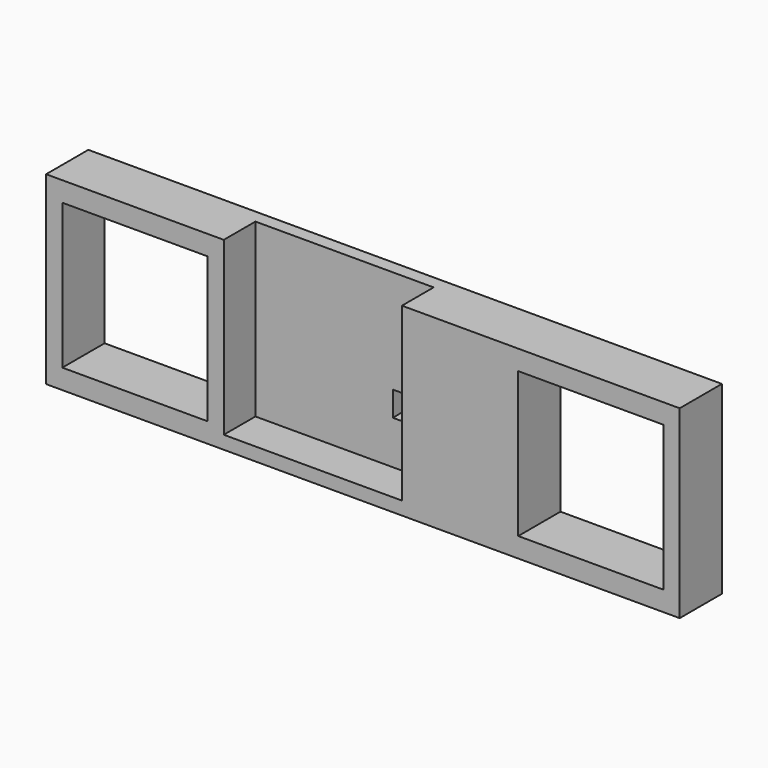
from build123d import *

# Parameters (mm, degrees)
F0_W     = 7.8232
F0_H     = 6.35
F0_W_2   = 69.85
F0_H_2   = 3.175
F0_W_3   = 55.9308
F0_H_3   = 69.85
F0_W_4   = 7.7978
F0_H_4   = 12.7
F0_W_5   = 85.725
F1_DEPTH = 25.4
F0_W_6   = 2.8702
F0_H_5   = 5.1918955931
F0_W_7   = 66.0908
F0_H_6   = 4.9097025247
F0_H_7   = 13.4315382606
F0_W_8   = 16.764
F0_H_8   = 0.762
F2_DEPTH = 6.35


with BuildPart() as f1:
    # F0 (on Front) → F1 (new body)
    with BuildSketch(Plane.XZ):
        with Locations((148.4884, 43.5362195122)):
            Rectangle(F0_W, F0_H)
        with Locations((109.6518, 43.5362195122)):
            Rectangle(F0_W_2, F0_H)
        with Locations((148.4884, 38.7737195122)):
            Rectangle(F0_W, F0_H_2)
        with Locations((46.7614, 43.5362195122)):
            Rectangle(F0_W_3, F0_H)
        with Locations((109.6518, 38.7737195122)):
            Rectangle(F0_W_2, F0_H_2)
        with Locations((148.4884, 2.2612195122)):
            Rectangle(F0_W, F0_H_3)
        with Locations((46.7614, 38.7737195122)):
            Rectangle(F0_W_3, F0_H_2)
        with Locations((148.4884, -34.2512804878)):
            Rectangle(F0_W, F0_H_2)
        with Locations((-70.8279, 43.5362195122)):
            Rectangle(F0_W_4, F0_H)
        Polygon((74.7268, -2.1837804878), (74.7268, 37.1862195122), (18.796, 37.1862195122), (18.796, 3.0081151053), (18.796, -2.1837804878), align=None)
        with Locations((109.6518, -34.2512804878)):
            Rectangle(F0_W_2, F0_H_2)
        with Locations((148.4884, -39.0137804878)):
            Rectangle(F0_W, F0_H)
        with Locations((-109.6518, 43.5362195122)):
            Rectangle(F0_W_2, F0_H)
        with Locations((-70.8279, 38.7737195122)):
            Rectangle(F0_W_4, F0_H_2)
        with Locations((46.7614, -8.5337804878)):
            Rectangle(F0_W_3, F0_H_4)
        with Locations((109.6518, -39.0137804878)):
            Rectangle(F0_W_2, F0_H)
        Polygon((18.796, -32.6637804878), (74.7268, -32.6637804878), (74.7268, -14.8837804878), (18.796, -14.8837804878), (18.796, -28.3153187484), align=None)
        with Locations((46.7614, -34.2512804878)):
            Rectangle(F0_W_3, F0_H_2)
        with Locations((-148.4884, 43.5362195122)):
            Rectangle(F0_W, F0_H)
        with Locations((-109.6518, 38.7737195122)):
            Rectangle(F0_W_2, F0_H_2)
        Polygon((-66.929, 2.7259220369), (-66.929, 37.1862195122), (-74.7268, 37.1862195122), (-74.7268, -2.1837804878), (-66.929, -2.1837804878), align=None)
        with Locations((46.7614, -39.0137804878)):
            Rectangle(F0_W_3, F0_H)
        with Locations((-148.4884, 38.7737195122)):
            Rectangle(F0_W, F0_H_2)
        with Locations((-24.0665, -39.0137804878)):
            Rectangle(F0_W_5, F0_H)
        Polygon((-74.7268, -32.6637804878), (-66.929, -32.6637804878), (-66.929, -28.3153187484), (-66.929, -14.8837804878), (-74.7268, -14.8837804878), align=None)
        with Locations((-70.8279, -34.2512804878)):
            Rectangle(F0_W_4, F0_H_2)
        with Locations((-148.4884, 2.2612195122)):
            Rectangle(F0_W, F0_H_3)
        with Locations((-70.8279, -8.5337804878)):
            Rectangle(F0_W_4, F0_H_4)
        with Locations((-70.8279, -39.0137804878)):
            Rectangle(F0_W_4, F0_H)
        with Locations((-109.6518, -34.2512804878)):
            Rectangle(F0_W_2, F0_H_2)
        with Locations((-148.4884, -34.2512804878)):
            Rectangle(F0_W, F0_H_2)
        with Locations((-109.6518, -39.0137804878)):
            Rectangle(F0_W_2, F0_H)
        with Locations((-148.4884, -39.0137804878)):
            Rectangle(F0_W, F0_H)
    extrude(amount=F1_DEPTH)

    # F0 (on Front) → F2 (join)
    with BuildSketch(Plane.XZ):
        with Locations((-24.0665, 43.5362195122)):
            Rectangle(F0_W_5, F0_H)
        with Locations((-70.8279, 43.5362195122)):
            Rectangle(F0_W_4, F0_H)
        with Locations((-24.0665, 38.7737195122)):
            Rectangle(F0_W_5, F0_H_2)
        with Locations((-70.8279, 38.7737195122)):
            Rectangle(F0_W_4, F0_H_2)
        Polygon((18.796, 3.0081151053), (18.796, 37.1862195122), (-66.929, 37.1862195122), (-66.929, 2.7259220369), (-0.8382, 2.7259220369), (-0.8382, 3.0081151053), (15.9258, 3.0081151053), align=None)
        with Locations((17.3609, 0.4121673088)):
            Rectangle(F0_W_6, F0_H_5)
        Polygon((18.796, -14.8837804878), (18.796, -2.1837804878), (15.9258, -2.1837804878), (15.9258, -2.9457804878), (15.9258, -14.8837804878), align=None)
        Polygon((-66.929, -32.6637804878), (18.796, -32.6637804878), (18.796, -28.3153187484), (15.9258, -28.3153187484), (-0.8382, -28.3153187484), (-66.929, -28.3153187484), align=None)
        with Locations((-24.0665, -34.2512804878)):
            Rectangle(F0_W_5, F0_H_2)
        with Locations((-33.8836, 0.2710707746)):
            Rectangle(F0_W_7, F0_H_6)
        Polygon((15.9258, -2.1837804878), (15.9258, 3.0081151053), (-0.8382, 3.0081151053), (-0.8382, 2.7259220369), (-0.8382, -2.1837804878), align=None)
        with Locations((17.3609, -21.5995496181)):
            Rectangle(F0_W_6, F0_H_7)
        with Locations((7.5438, -2.5647804878)):
            Rectangle(F0_W_8, F0_H_8)
        Polygon((-0.8382, -2.1837804878), (-66.929, -2.1837804878), (-66.929, -14.8837804878), (-0.8382, -14.8837804878), (-0.8382, -2.9457804878), align=None)
        with Locations((7.5438, -21.5995496181)):
            Rectangle(F0_W_8, F0_H_7)
        with Locations((-33.8836, -21.5995496181)):
            Rectangle(F0_W_7, F0_H_7)
    extrude(amount=F2_DEPTH)


solid = f1.part
